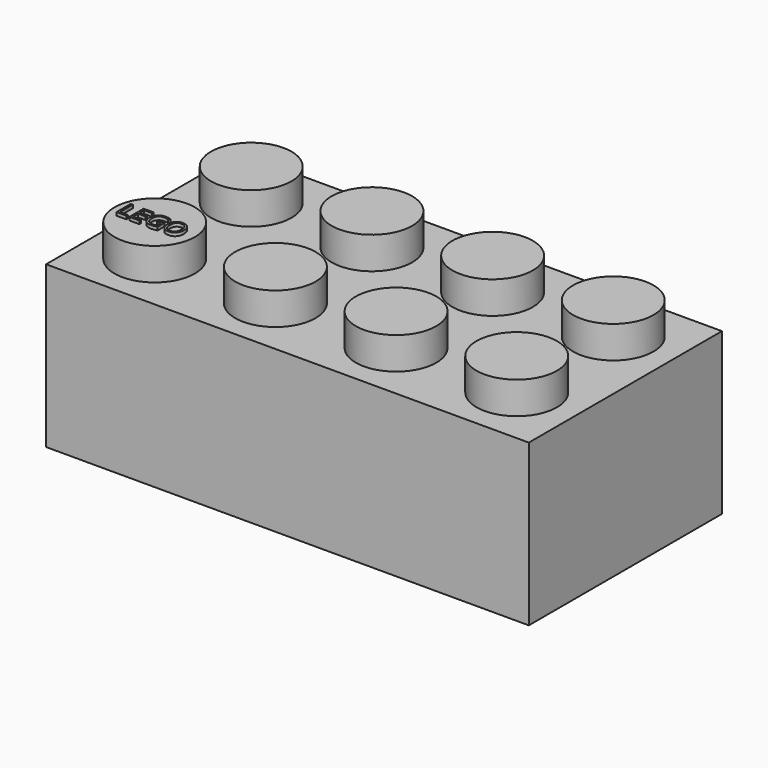
from build123d import *

# Parameters (mm, degrees)
F0_W         = 30
F0_H         = 15
F1_DEPTH     = 10
F2_R         = 2.5
F3_DEPTH     = 2
F4_W         = 29.2
F4_H         = 14.2
F4_R         = 2.5
F4_R_2       = 2.25
F5_DEPTH     = 8
F6_TEXT_SIZE = 1.5469212641
F7_DEPTH     = 0.2


# Not quite as in the source:
# - Text() gives the source's letters only with a copy of the font that has no kerning and outlines rounded to 1/6400 em; it was checked with that copy


with BuildPart() as f1:
    # F0 (on Top) → F1 (new body)
    with BuildSketch(Plane.XY):
        with Locations((2.3510786705, 0.4816347342)):
            Rectangle(F0_W, F0_H)
    extrude(amount=F1_DEPTH)

    # F2 (on face) → F3 (join)
    with BuildSketch(Plane.XY.offset(10)):
        with Locations((-8.8989213295, 4.2316347342)):
            Circle(F2_R)
        with Locations((-1.3989213295, 4.2316347342)):
            Circle(F2_R)
        with Locations((6.1010786705, 4.2316347342)):
            Circle(F2_R)
        with Locations((13.6010786705, 4.2316347342)):
            Circle(F2_R)
        with Locations((13.6010786705, -3.2683652658)):
            Circle(F2_R)
        with Locations((6.1010786705, -3.2683652658)):
            Circle(F2_R)
        with Locations((-1.3989213295, -3.2683652658)):
            Circle(F2_R)
        with Locations((-8.8989213295, -3.2683652658)):
            Circle(F2_R)
    extrude(amount=F3_DEPTH)

    # F4 (on face) → F5 (cut)
    with BuildSketch(Plane(origin=(0, 0, 0), x_dir=(1, 0, 0), z_dir=(0, 0, -1))):
        with Locations((2.3510786705, -0.4816347342)):
            Rectangle(F4_W, F4_H)
        with Locations((-7.6489213295, -0.4816347342)):
            Circle(F4_R, mode=Mode.SUBTRACT)
        with Locations((2.3510786705, -0.4816347342)):
            Circle(F4_R, mode=Mode.SUBTRACT)
        with Locations((12.3510786705, -0.4816347342)):
            Circle(F4_R, mode=Mode.SUBTRACT)
        with Locations((-7.6489213295, -0.4816347342)):
            Circle(F4_R_2)
        with Locations((2.3510786705, -0.4816347342)):
            Circle(F4_R_2)
        with Locations((12.3510786705, -0.4816347342)):
            Circle(F4_R_2)
    extrude(amount=-F5_DEPTH, mode=Mode.SUBTRACT)

    # F6 (on face) → F7 (join)
    with BuildSketch(Plane.XY.offset(12)):
        with Locations((-10.916088652, -3.903013022)):
            Text('LEGO', F6_TEXT_SIZE, font='Open Sans', text_align=(TextAlign.LEFT, TextAlign.BOTTOM))
    extrude(amount=F7_DEPTH)


solid = f1.part
